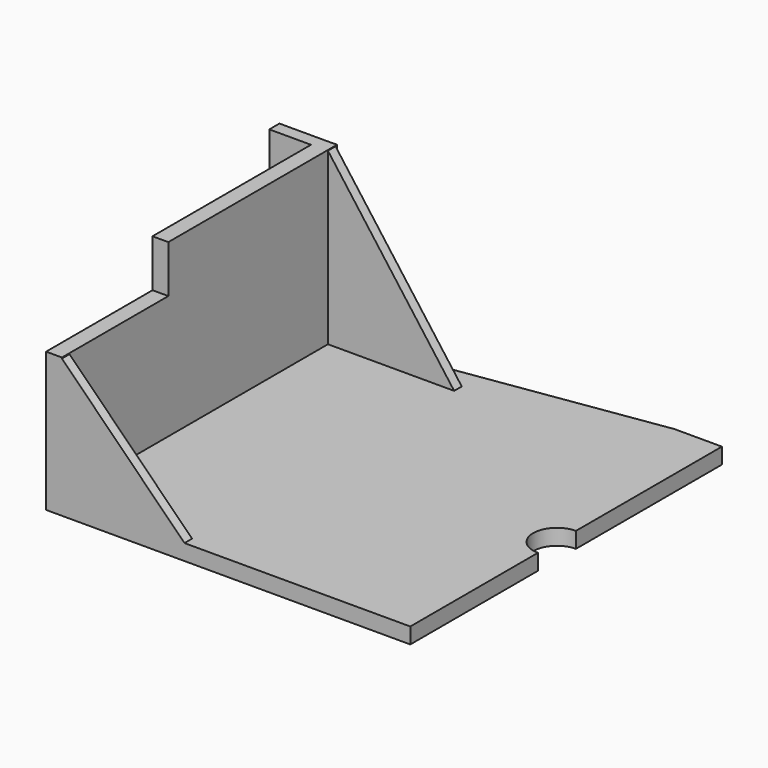
from build123d import *

# Parameters (mm, degrees)
F1_DEPTH     = 5
F2_SIZE2     = 100
F2_SIZE      = 15
F3_W         = 5
F3_H         = 108
F4_DEPTH     = 54
F4_FACE_W    = 5
F4_FACE_H    = 54
F5_ANGLE     = 7.9800839779
F6_W         = 42
F6_H         = 15
F7_DEPTH     = 25
F8_W         = 7.5
F8_H         = 11
F9_DEPTH     = 16
F10_T4_DEPTH = 91.0129088322
F11_R        = 3
F12_W        = 18
F12_H        = 4
F13_DEPTH    = 59
F14_W        = 40
F14_H        = 3
F15_DEPTH    = 38.7
F16_DEPTH    = 15.2
F17_T1_DEPTH = 208.7346390373
F17_T6_DEPTH = 207.8673195186
F18_T4_DEPTH = 299.280483699


# Not quite as in the source:
# - a fillet or chamfer that OpenCascade refuses, or shapes differently, is made with other operations: its cross-section is extruded or revolved along the edge and cut away or added


with BuildPart() as f1:
    # F0 (on Top) → F1 (new body)
    with BuildSketch(Plane.XY):
        with BuildLine():
            Line((57.5, 3.8800953701), (57.5, 61.5))
            Line((57.5, 61.5), (-57.5, 61.5))
            Line((-57.5, 61.5), (-57.5, -61.5))
            Line((-57.5, -61.5), (57.5, -61.5))
            Line((57.5, -61.5), (57.5, -11.1199046299))
            ThreePointArc((57.5, -11.1199046299), (50, -3.6199046299), (57.5, 3.8800953701))
        make_face()
    extrude(amount=F1_DEPTH)

    # F2
    f2_edges = [f1.edges().sort_by_distance(p)[0] for p in [
        (-57.5, 61.5, 2.5),
    ]]
    f2_side = f1.faces().sort_by_distance((-57.5, 0, 2.5))[0]
    chamfer(f2_edges, length=F2_SIZE, length2=F2_SIZE2, reference=f2_side)

    # F3 (on face) → F4 (join)
    with BuildSketch(Plane.XY.offset(5)):
        with Locations((-55, -7.5)):
            Rectangle(F3_W, F3_H)
    extrude(amount=F4_DEPTH)

    # F4_face (on face) → F5 (revolve)
    with BuildSketch(Plane(origin=(-55, 46.5, 32), x_dir=(-1, 0, 0), z_dir=(0, 1, 0))):
        Rectangle(F4_FACE_W, F4_FACE_H)
    revolve(axis=Axis((-57.5, 46.5, 32), (0, 0, 1)), revolution_arc=F5_ANGLE)

    # F6 (on face) → F7 (cut)
    with BuildSketch(Plane.YZ.offset(-52.5)):
        with Locations((-40.5, 51.5)):
            Rectangle(F6_W, F6_H)
    extrude(amount=-F7_DEPTH, mode=Mode.SUBTRACT)

    # F8 (on face) → F9 (join)
    with BuildSketch(Plane(origin=(-57.5, 0, 0), x_dir=(0, -1, 0), z_dir=(-1, 0, 0))):
        with Locations((23.25, 5.5)):
            Rectangle(F8_W, F8_H)
    extrude(amount=F9_DEPTH)

    # F10: chamfer of 16.1 x 6.2 on 1 edges, made by hand


with BuildPart() as f10_tool2:
    # F10_s3 → F10_t4 (new body)
    with BuildSketch(Plane.XZ.offset(68.7564544161)):
        Polygon((-57.4, 11), (-73.5, 4.8), (-73.5, 11), align=None)
    extrude(amount=-F10_T4_DEPTH)

    split(bisect_by=Plane.YZ.offset(-57.5), keep=Keep.BOTTOM)


with BuildPart() as f1_1:
    add(f1.part)

    # F10_t1: cut F10_tool2
    add(f10_tool2.part, mode=Mode.SUBTRACT)

    # F11
    f11_edges = [f1_1.edges().sort_by_distance(p)[0] for p in [
        (-65.5, -27, 7.880745),
        (-65.5, -19.5, 7.880745),
    ]]
    fillet(f11_edges, radius=F11_R)

    # F12 (on Top) → F13 (join)
    with BuildSketch(Plane.XY):
        with Locations((-61.6593700051, 45.0587611198)):
            Rectangle(F12_W, F12_H)
    extrude(amount=F13_DEPTH)

    # F14 (on face) → F15 (join)
    with BuildSketch(Plane.XY.offset(5)):
        with Locations((-32.5, -60)):
            Rectangle(F14_W, F14_H)
        with Locations((-32.5, 45)):
            Rectangle(F14_W, F14_H)
    extrude(amount=F15_DEPTH)

    # F16 (add): a face of the model
    f16_faces = [f1_1.faces().sort_by_distance(p)[0] for p in [
        (-32.5, 45, 43.7),
    ]]
    extrude(f16_faces, amount=F16_DEPTH)

    # F17: chamfer of 40 on 2 edges, made by hand

    # F17_s2 → F17_t1 (cut)
    with BuildSketch(Plane.XZ.offset(-149.3673195186)):
        Polygon((-52.5, 58.9), (-12.5, 18.9), (-12.5, 58.9), align=None)
    extrude(amount=F17_T1_DEPTH, mode=Mode.SUBTRACT)


with BuildPart() as f17_tool4:
    # F17_s5 → F17_t6 (new body)
    with BuildSketch(Plane.XZ.offset(164.3673195186)):
        Polygon((-52.5, 43.7), (-12.5, 3.7), (-12.5, 43.7), align=None)
    extrude(amount=-F17_T6_DEPTH)

    split(bisect_by=Plane.XY.offset(5), keep=Keep.TOP)


with BuildPart() as f1_2:
    add(f1_1.part)

    # F17_t3: cut F17_tool4
    add(f17_tool4.part, mode=Mode.SUBTRACT)

    # F18: chamfer of 14.1 x 57 on 1 edges, made by hand


with BuildPart() as f18_tool2:
    # F18_s3 → F18_t4 (new body)
    with BuildSketch(Plane.XZ.offset(-194.6402418495)):
        Polygon((-52.8050865276, 59.2050865276), (-12.5, 4.8), (-12.5, 18.9), align=None)
    extrude(amount=F18_T4_DEPTH)

    split(bisect_by=Plane.XY.offset(5), keep=Keep.TOP)

    split(bisect_by=Plane.YZ.offset(-52.5), keep=Keep.TOP)


with BuildPart() as f1_3:
    add(f1_2.part)

    # F18_t1: cut F18_tool2
    add(f18_tool2.part, mode=Mode.SUBTRACT)


solid = f1_3.part
